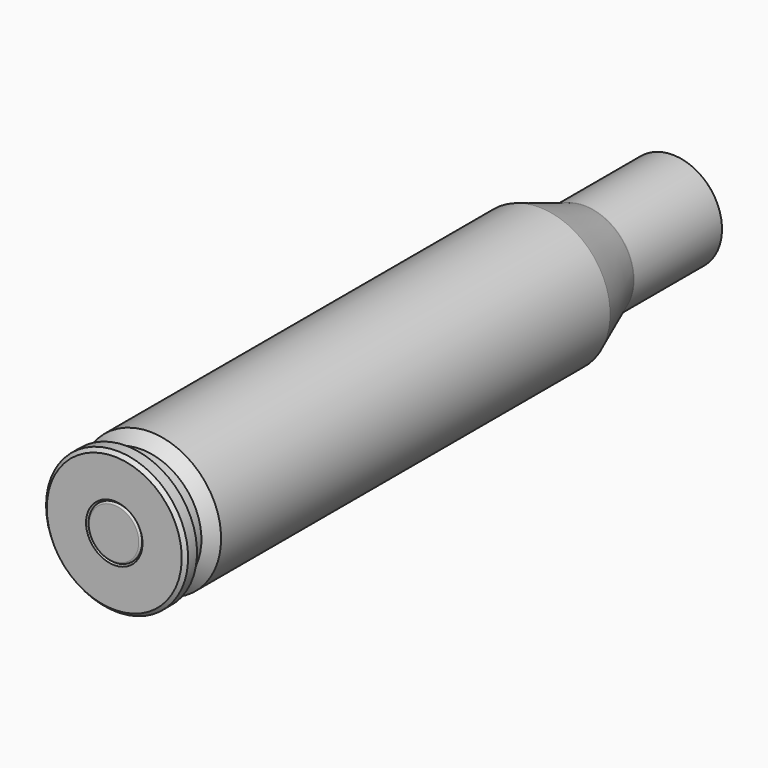
from build123d import *

# Parameters (mm, degrees)
F3_DEPTH = 5.3848
F4_R     = 0.254
F5_SIZE  = 0.508
F6_R     = 3.175
F7_DEPTH = 12.7


# Not quite as in the source:
# - a fillet or chamfer that OpenCascade refuses, or shapes differently, is made with other operations: its cross-section is extruded or revolved along the edge and cut away or added


with BuildPart() as f1:
    # F0 (on Top) → F1 (revolve)
    with BuildSketch(Plane.XY):
        Polygon((-19.1289222062, -69.1020740439), (-15.3252963252, -69.1020740439), (-15.3252963252, 26.1417003232), (-21.4466963252, 26.1417003232), (-22.4372963252, 26.1417003232), (-22.4372963252, 10.0381003232), (-25.5360963252, 1.9012442353), (-25.5360963252, -68.0084118526), (-23.9612963252, -69.5832118526), (-23.9612963252, -72.3429557647), (-25.5360963252, -72.3429557647), (-25.5360963252, -74.4511557647), (-19.1289222062, -74.4511557647), align=None)
    revolve(axis=Axis((-15.3252963252, -24.1547277207, 0), (0, 1, 0)))

    # F2: chamfer of 0.254 on 3 edges, made by hand

    # F2_s1 → F2_t2 (revolve)
    with BuildSketch(Plane.XY):
        Polygon((-22.4372963252, 10.0848293801), (-22.4539271766, 9.9944308884), (-22.4372963252, 10.0381003232), align=None)
    revolve(axis=Axis((-15.3252963252, 10.0381003232, 0), (0, 1, 0)))

    # F2_s3 → F2_t4 (revolve, cut)
    with BuildSketch(Plane.XY):
        Polygon((-19.3829222062, -74.4511557647), (-19.1289222062, -74.1971557647), (-19.1289222062, -74.4511557647), align=None)
    revolve(axis=Axis((-15.3252963252, -74.4511557647, 0), (0, 1, 0)), mode=Mode.SUBTRACT)

    # F2_s5 → F2_t6 (revolve, cut)
    with BuildSketch(Plane.XY):
        Polygon((-22.1832963252, 26.1417003232), (-22.4372963252, 25.8877003232), (-22.4372963252, 26.1417003232), align=None)
    revolve(axis=Axis((-15.3252963252, 26.1417003232, 0), (0, 1, 0)), mode=Mode.SUBTRACT)

    # F3 (add): a face of the model
    f3_faces = [f1.faces().sort_by_distance(p)[0] for p in [
        (-15.3252963252, -69.1020740439, 0),
    ]]
    extrude(f3_faces, amount=F3_DEPTH)

    # F4
    f4_edges = [f1.edges().sort_by_distance(p)[0] for p in [
        (-11.52167, -74.486874, 0),
    ]]
    fillet(f4_edges, radius=F4_R)

    # F5
    f5_edges = [f1.edges().sort_by_distance(p)[0] for p in [
        (-5.114496, -74.451156, 0),
    ]]
    chamfer(f5_edges, length=F5_SIZE)

    # F6 (on face) → F7 (cut)
    with BuildSketch(Plane(origin=(0, 26.1417003232, 0), x_dir=(-1, 0, 0), z_dir=(0, 1, 0))):
        with Locations((15.3252963252, 0)):
            Circle(F6_R)
    extrude(amount=-F7_DEPTH, mode=Mode.SUBTRACT)


solid = f1.part
